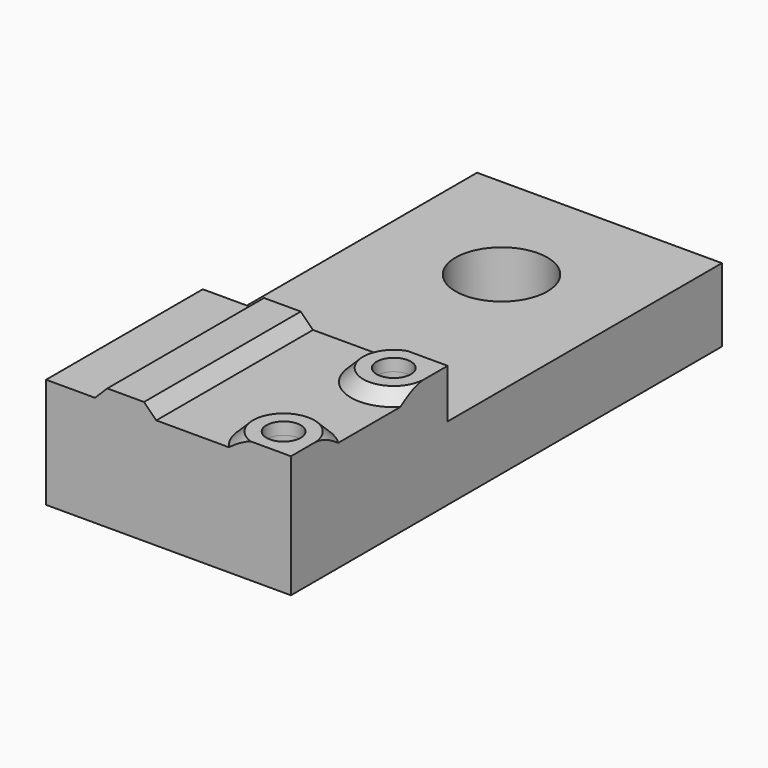
from build123d import *

# Parameters (mm, degrees)
F0_W      = 20
F0_H      = 44
F1_DEPTH  = 10
F2_R      = 1.4
F3_DEPTH  = 10.001
F5_DEPTH  = 20.001
F6_R      = 2.25
F7_DEPTH  = 6.001
F8_R      = 3.75
F9_DEPTH  = 4
F10_W     = 3
F10_H     = 16
F10_R     = 1.4
F11_DEPTH = 1
F12_SIZE  = 0.99999


# Not quite as in the source:
# - a fillet or chamfer is up to 0.001 mm smaller than in the source, because OpenCascade refuses the exact size
# - a pattern or mirror of a feature is missing from the dataset's text; its kind, count and spacing are read off the source's solid


with BuildPart() as f1:
    # F0 (on Top) → F1 (new body)
    with BuildSketch(Plane.XY):
        Rectangle(F0_W, F0_H)
    extrude(amount=F1_DEPTH)

    # F2 (on face) → F3 (cut, through all)
    with BuildSketch(Plane.XY.offset(10)):
        with Locations((7.5, -19.625)):
            Circle(F2_R)
        with Locations((7.5, -8.375)):
            Circle(F2_R)
    extrude(amount=-F3_DEPTH, mode=Mode.SUBTRACT)

    # F4 (on face) → F5 (cut, through all)
    with BuildSketch(Plane(origin=(-10, 0, 0), x_dir=(0, -1, 0), z_dir=(-1, 0, 0))):
        Polygon((6, 9), (22, 9), (22, 10), (-22, 10), (-22, 6), (6, 6), align=None)
    extrude(amount=-F5_DEPTH, mode=Mode.SUBTRACT)

    # F6 (on face) → F7 (cut, through all)
    with BuildSketch(Plane.XY.offset(6)):
        with Locations((0, 12)):
            Circle(F6_R)
    extrude(amount=-F7_DEPTH, mode=Mode.SUBTRACT)

    # F8 (on face) → F9 (cut)
    with BuildSketch(Plane.XY.offset(6)):
        with Locations((0, 12)):
            Circle(F8_R)
    extrude(amount=-F9_DEPTH, mode=Mode.SUBTRACT)

    # F10 (on face) → F11 (join)
    with BuildSketch(Plane.XY.offset(9)):
        with Locations((-3.5, -14)):
            Rectangle(F10_W, F10_H)
        with BuildLine():
            Line((10, -22), (10, -17.1755102572))
            ThreePointArc((10, -17.1755102572), (5.0874948755, -17.0892912185), (4.9291295248, -22))
            Line((4.9291295248, -22), (10, -22))
        make_face()
        with Locations((7.5, -19.625)):
            Circle(F10_R, mode=Mode.SUBTRACT)
    f11 = extrude(amount=F11_DEPTH)

    # F11_copies: F11 across plane
    add(f11.mirror(Plane(origin=(-6e-06, -13.999993, 0), x_dir=(0, 0, 1), z_dir=(0, 1, 0))))

    # F12 (size 1 in the source; OpenCascade refuses exactly that, so slightly less here)
    f12_edges = [f1.edges().sort_by_distance(p)[0] for p in [
        (5.087495, -10.910695, 10),
        (5.087495, -17.089291, 10),
        (-5, -14, 9),
        (-2, -14, 9),
    ]]
    chamfer(f12_edges, length=F12_SIZE)


solid = f1.part
